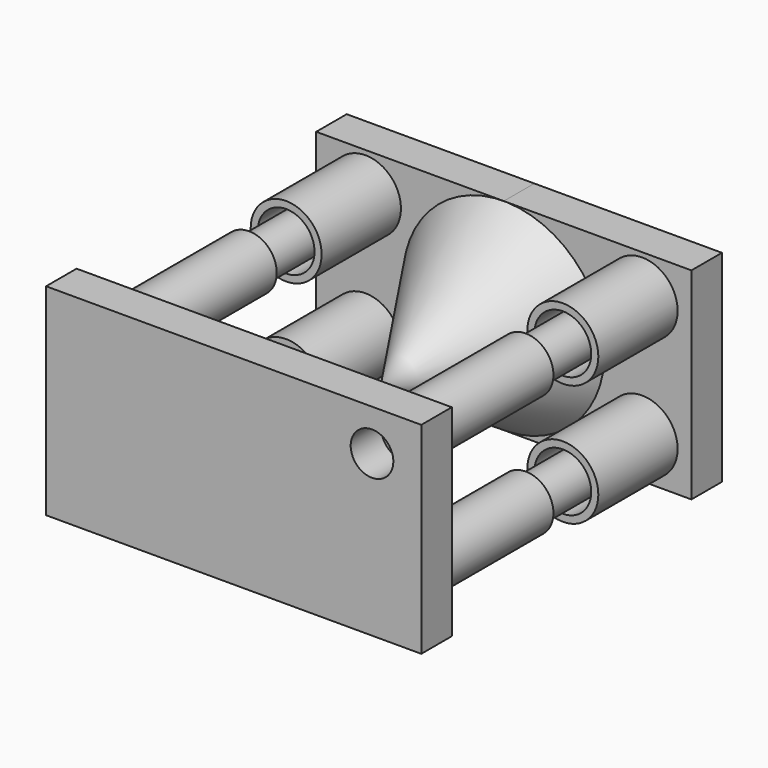
from build123d import *

# Parameters (mm, degrees)
F2_T      = -0.254
F3_W      = 18.7457744032
F3_H      = 20.1506689191
F4_DEPTH  = 3.81
F5_R      = 2.130532704
F6_DEPTH  = 29.929663986
F5_R_2    = 3.5450449464
F5_R_3    = 2.8368433818
F8_DEPTH  = 9.906
F9_R      = 2.7648346721
F10_DEPTH = 15.3924
F14_T     = -0.254
F15_W     = 18.7452
F15_H     = 20.1422
F15_R     = 2.130532704
F16_DEPTH = 3.81


# Not quite as in the source:
# - the program builds the solid bodies; features that only make, move or delete a surface that nothing else refers to are left out


with BuildPart() as f1:
    # F0 (on Top) → F1 (revolve)
    with BuildSketch(Plane.XY):
        Polygon((-10.0753344595, 55.7106658816), (0, 40.3013341129), (0, 55.7106658816), align=None)
    revolve(axis=Axis((0, 48.0059999973, 0), (0, 1, 0)))

    # F2
    f2_openings = [f1.faces().sort_by_distance(p)[0] for p in [
        (0, 55.710666, 0),
    ]]
    offset(amount=F2_T, openings=f2_openings)


with BuildPart() as f1b:
    # F0 (on Top) → F1, piece 2 (revolve)
    with BuildSketch(Plane.XY):
        Polygon((-10.0753344595, 25.7810018957), (0, 25.7810018957), (0, 40.3013341129), align=None)
    revolve(axis=Axis((0, 48.0059999973, 0), (0, 1, 0)))

    # F14
    f14_openings = [f1b.faces().sort_by_distance(p)[0] for p in [
        (0, 25.781002, 0),
    ]]
    offset(amount=F14_T, openings=f14_openings)


with BuildPart() as f4:
    # F3 (on face) → F4 (new body)
    with BuildSketch(Plane(origin=(0, 55.7106658816, 0), x_dir=(-1, 0, 0), z_dir=(0, 1, 0))):
        with Locations((-9.3728872016, 0)):
            Rectangle(F3_W, F3_H)
    extrude(amount=F4_DEPTH)

    # F5 (on face) → F8 (join)
    with BuildSketch(Plane.XZ.offset(-55.7106658816)):
        with Locations((13.8234719634, 6.072612945)):
            Circle(F5_R_2)
        with Locations((13.8234719634, 6.072612945)):
            Circle(F5_R_3, mode=Mode.SUBTRACT)
    extrude(amount=F8_DEPTH)


with BuildPart() as f6:
    # F5 (on face) → F6 (new body, through all)
    with BuildSketch(Plane.XZ.offset(-55.7106658816)):
        with Locations((13.8234719634, 6.072612945)):
            Circle(F5_R)
    extrude(amount=F6_DEPTH)


with BuildPart() as f10:
    # F9 (on face) → F10 (new body)
    with BuildSketch(Plane.XZ.offset(-25.7810018957)):
        with Locations((13.8234719634, 6.072612945)):
            Circle(F9_R)
    extrude(amount=-F10_DEPTH)


with BuildPart() as f11_1:
    # F11: instance of F4
    add(f4.part.mirror(Plane(origin=(0, 57.6156658816, 0), x_dir=(0, -1, 0), z_dir=(-1, 0, 0))))


with BuildPart() as f11_2:
    # F11: instance of F6
    add(f6.part.mirror(Plane(origin=(0, 57.6156658816, 0), x_dir=(0, -1, 0), z_dir=(-1, 0, 0))))


with BuildPart() as f11_3:
    # F11: instance of F10
    add(f10.part.mirror(Plane(origin=(0, 57.6156658816, 0), x_dir=(0, -1, 0), z_dir=(-1, 0, 0))))


with BuildPart() as f12_1:
    # F12: instance of F6
    add(f6.part.mirror(Plane.XY))


with BuildPart() as f12_2:
    # F12: instance of F10
    add(f10.part.mirror(Plane.XY))


with BuildPart() as f12_3:
    # F12: instance of F4
    add(f4.part.mirror(Plane.XY))


with BuildPart() as f13_1:
    # F13: instance of F11_1
    add(f11_1.part.mirror(Plane.XY))


with BuildPart() as f13_2:
    # F13: instance of F11_2
    add(f11_2.part.mirror(Plane.XY))


with BuildPart() as f13_3:
    # F13: instance of F11_3
    add(f11_3.part.mirror(Plane.XY))


with BuildPart() as f16:
    # F15 (on face) → F16 (new body)
    with BuildSketch(Plane.XZ.offset(-25.7810018957)):
        with Locations((9.3726, 0.1313106309)):
            Rectangle(F15_W, F15_H)
        with Locations((13.8234719634, 6.072612945)):
            Circle(F15_R, mode=Mode.SUBTRACT)
        with Locations((-9.3726, 0.1313106309)):
            Rectangle(F15_W, F15_H)
    extrude(amount=F16_DEPTH)


solid = Compound([f1.part, f1b.part, f4.part, f6.part, f10.part, f11_1.part, f11_2.part, f11_3.part, f12_1.part, f12_2.part, f12_3.part, f13_1.part, f13_2.part, f13_3.part, f16.part])
